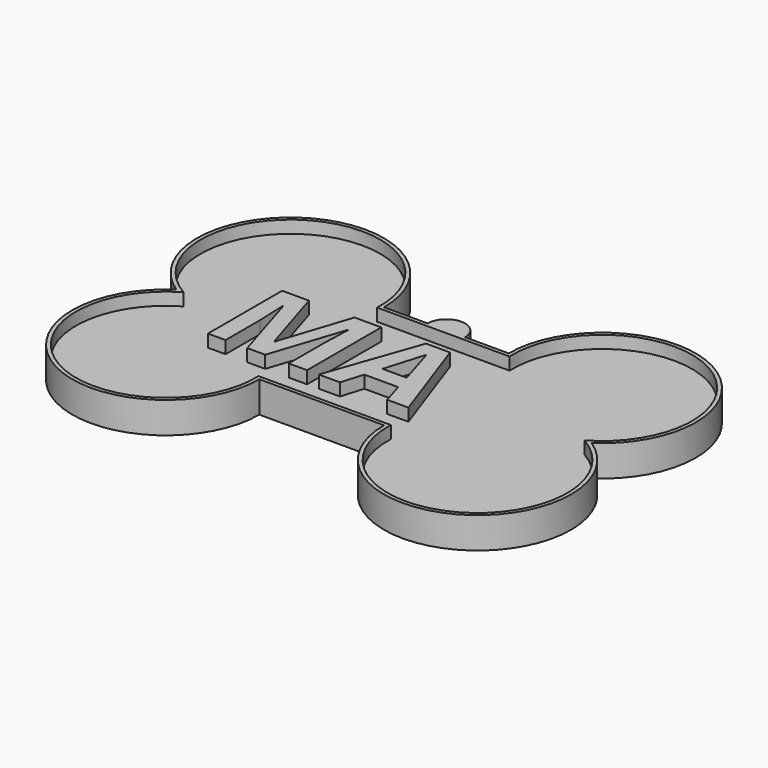
from build123d import *

# Parameters (mm, degrees)
F1_DEPTH = 3
F3_DEPTH = 2
F5_DEPTH = 2
F6_DEPTH = 2


# Not quite as in the source:
# - a feature of the source that left no trace in its solid (it failed there, or was rolled back) is left out


with BuildPart() as f1:
    # F0 (on Top) → F1 (new body)
    with BuildSketch(Plane.XY):
        with BuildLine():
            Line((-3, 12.5), (-10, 12.5))
            ThreePointArc((-10, 12.5), (-32.0931858273, 25.7169101843), (-33.2915619759, 0))
            ThreePointArc((-33.2915619759, 0), (-32.0931858273, -25.7169101843), (-10, -12.5))
            Line((-10, -12.5), (10, -12.5))
            ThreePointArc((10, -12.5), (32.0931858273, -25.7169101843), (33.2915619759, 0))
            ThreePointArc((33.2915619759, 0), (32.0931858273, 25.7169101843), (10, 12.5))
            Line((10, 12.5), (3, 12.5))
            ThreePointArc((3, 12.5), (0, 15.5), (-3, 12.5))
        make_face()
    extrude(amount=F1_DEPTH)

    # F2 (on face) → F3 (join)
    with BuildSketch(Plane.XY.offset(3)):
        with BuildLine():
            ThreePointArc((33.2915619759, 0), (32.0931858273, 25.7169101843), (10, 12.5))
            Line((10, 12.5), (3, 12.5))
            ThreePointArc((3, 12.5), (0, 15.5), (-3, 12.5))
            Line((-3, 12.5), (-10, 12.5))
            ThreePointArc((-10, 12.5), (-32.0931858273, 25.7169101843), (-33.2915619759, 0))
            ThreePointArc((-33.2915619759, 0), (-32.0931858273, -25.7169101843), (-10, -12.5))
            Line((-10, -12.5), (10, -12.5))
            ThreePointArc((10, -12.5), (32.0931858273, -25.7169101843), (33.2915619759, 0))
        make_face()
        with BuildLine():
            ThreePointArc((-10.6125054301, -11.9), (-31.9642656137, -25.1039281362), (-32.1491258207, 0))
            ThreePointArc((-32.1491258207, 0), (-31.9642656137, 25.1039281362), (-10.6125054301, 11.9))
            Line((-10.6125054301, 11.9), (0, 11.9))
            Line((0, 11.9), (10.6125054301, 11.9))
            ThreePointArc((10.6125054301, 11.9), (31.9642656137, 25.1039281362), (32.1491258207, 0))
            ThreePointArc((32.1491258207, 0), (31.9642656137, -25.1039281362), (10.6125054301, -11.9))
            Line((10.6125054301, -11.9), (-10.6125054301, -11.9))
        make_face(mode=Mode.SUBTRACT)
    extrude(amount=F3_DEPTH)

    # F4 (on face) → F5 (join)
    with BuildSketch(Plane.XY.offset(3)):
        with BuildLine():
            Line((-20.0455729167, 4.8259567143), (-16.46484375, -6.8407099524))
            Line((-16.46484375, -6.8407099524), (-13.57421875, -6.8407099524))
            Line((-13.57421875, -6.8407099524), (-9.7395833333, 4.8064254643))
            Line((-9.7395833333, 4.8064254643), (-9.6484375, 4.8064254643))
            add(Edge.make_bspline(
                [(-9.78515625, 1.3493942143), (-9.7688802083, 2.000435881), (-9.6484375, 4.8064254643)],
                knots=[0, 0, 0, 1, 1, 1], degree=2))
            add(Edge.make_bspline(
                [(-9.8014322917, 0.2003056726), (-9.8014322917, 0.6983525476), (-9.78515625, 1.3493942143)],
                knots=[0, 0, 0, 1, 1, 1], degree=2))
            Line((-9.8014322917, 0.2003056726), (-9.8014322917, -6.8407099524))
            Line((-9.8014322917, -6.8407099524), (-6.8619791667, -6.8407099524))
            Line((-6.8619791667, -6.8407099524), (-6.8619791667, 8.0323369226))
            Line((-6.8619791667, 8.0323369226), (-11.15234375, 8.0323369226))
            Line((-11.15234375, 8.0323369226), (-14.8860677083, -3.341360994))
            Line((-14.8860677083, -3.341360994), (-14.9479166667, -3.341360994))
            Line((-14.9479166667, -3.341360994), (-18.466796875, 8.0323369226))
            Line((-18.466796875, 8.0323369226), (-22.7604166667, 8.0323369226))
            Line((-22.7604166667, 8.0323369226), (-22.7604166667, -6.8407099524))
            Line((-22.7604166667, -6.8407099524), (-19.94140625, -6.8407099524))
            Line((-19.94140625, -6.8407099524), (-19.94140625, 0.076607756))
            add(Edge.make_bspline(
                [(-20.13671875, 4.8259567143), (-19.94140625, 1.268014006), (-19.94140625, 0.076607756)],
                knots=[0, 0, 0, 1, 1, 1], degree=2))
            Line((-20.13671875, 4.8259567143), (-20.0455729167, 4.8259567143))
        make_face()
    extrude(amount=F5_DEPTH)

    # F4 (on face) → F6 (join)
    with BuildSketch(Plane.XY.offset(3)):
        Polygon((4.9088541667, -3.2990432857), (5.986328125, -6.8407099524), (9.384765625, -6.8407099524), (4.1145833333, 8.094185881), (0.2604166667, 8.094185881), (-4.990234375, -6.8407099524), (-1.591796875, -6.8407099524), (-0.5143229167, -3.2990432857), align=None)
        with BuildLine():
            add(Edge.make_bspline(
                [(4.1536458333, -0.655814119), (2.6595052083, 4.1553837976), (2.470703125, 4.7868942143)],
                knots=[0, 0, 0, 1, 1, 1], degree=2))
            Line((4.1536458333, -0.655814119), (0.2799479167, -0.655814119))
            add(Edge.make_bspline(
                [(2.2005208333, 5.7829879643), (1.865234375, 4.480904631), (0.2799479167, -0.655814119)],
                knots=[0, 0, 0, 1, 1, 1], degree=2))
            add(Edge.make_bspline(
                [(2.470703125, 4.7868942143), (2.2819010417, 5.418404631), (2.2005208333, 5.7829879643)],
                knots=[0, 0, 0, 1, 1, 1], degree=2))
        make_face(mode=Mode.SUBTRACT)
    extrude(amount=F6_DEPTH)


solid = f1.part
